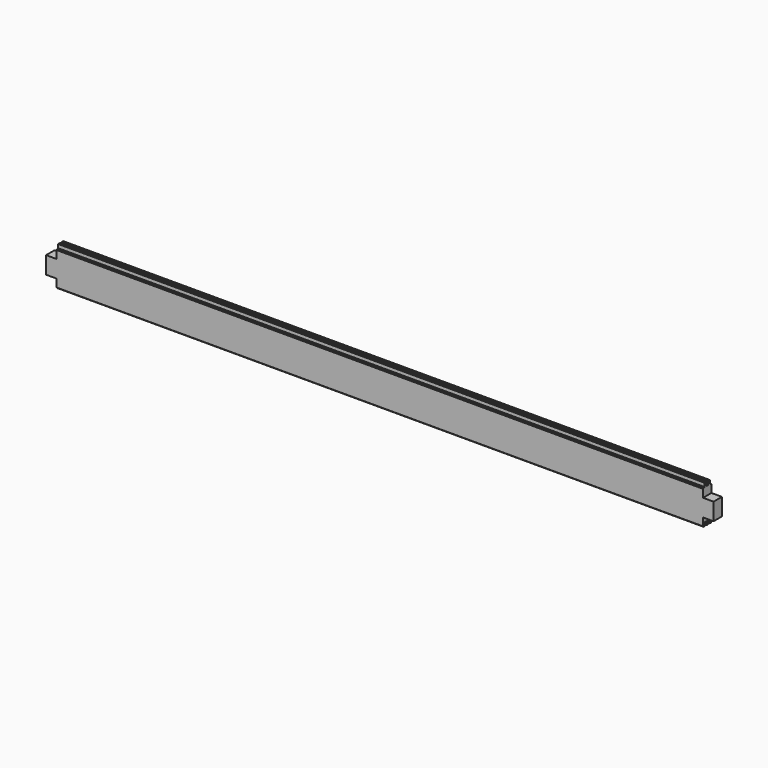
from build123d import *

# Parameters (mm, degrees)
F1_W     = 40
F1_H     = 33
F3_DEPTH = 1275
F2_W     = 80
F2_H     = 100
F4_DEPTH = 25


with BuildPart() as f3:
    # F1 (on Right) → F3 (new body, symmetric)
    with BuildSketch(Plane.YZ):
        Polygon((20, 33), (20, 63), (17, 66), (12, 66), (12, 80), (4, 80), (4, 66), (-4, 66), (-4, 80), (-12, 80), (-12, 66), (-17, 66), (-20, 63), (-20, 33), align=None)
        with Locations((0, 16.5)):
            Rectangle(F1_W, F1_H)
        with Locations((0, -16.5)):
            Rectangle(F1_W, F1_H)
        Polygon((20, -63), (20, -33), (-20, -33), (-20, -63), (-17, -66), (-12, -66), (-12, -52), (-4, -52), (-4, -66), (4, -66), (4, -52), (12, -52), (12, -66), (17, -66), align=None)
    extrude(amount=F3_DEPTH, both=True)

    # F2 (on Front) → F4 (cut, symmetric)
    with BuildSketch(Plane.XZ):
        with Locations((-1275, 83)):
            Rectangle(F2_W, F2_H)
        with Locations((-1275, -83)):
            Rectangle(F2_W, F2_H)
        with Locations((1275, 83)):
            Rectangle(F2_W, F2_H)
        with Locations((1275, -83)):
            Rectangle(F2_W, F2_H)
    extrude(amount=F4_DEPTH, both=True, mode=Mode.SUBTRACT)


solid = f3.part
